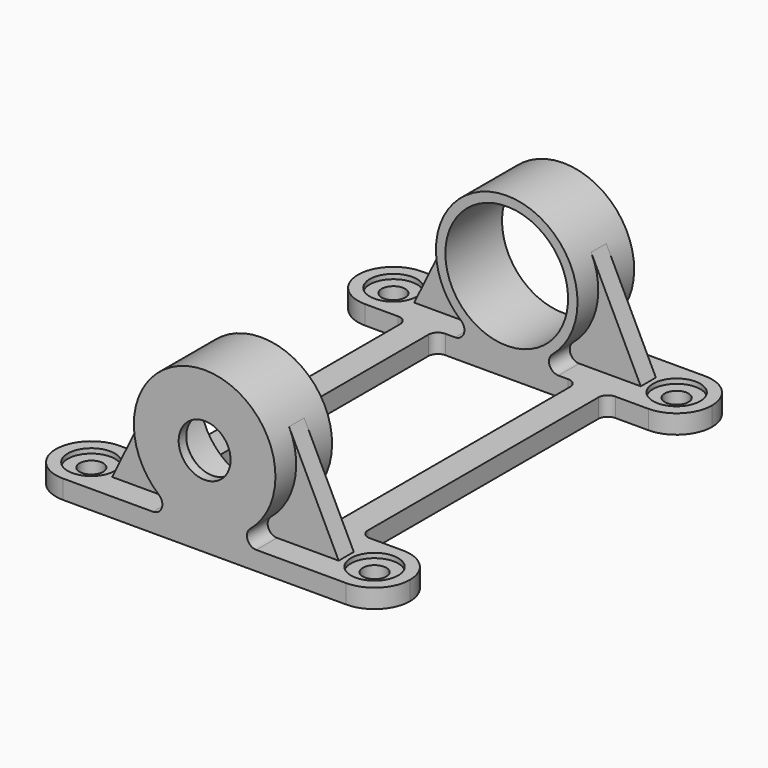
from build123d import *

# Parameters (mm, degrees)
F3_DEPTH       = 7.5
F4_R           = 7.49999
F6_D           = 5
F6_CBORE_D     = 10
F6_CBORE_DEPTH = 1
F8_DEPTH       = 2
F12_R          = 13
F13_DEPTH      = 92
F14_R          = 5.5
F15_DEPTH      = 95.001
F16_W          = 6
F16_H          = 4
F17_DEPTH      = 65
F18_R          = 2
F19_SIZE       = 1


# Not quite as in the source:
# - a fillet or chamfer is up to 0.001 mm smaller than in the source, because OpenCascade refuses the exact size


with BuildPart() as f3:
    # F2 (on Front) → F3 (new body, symmetric)
    with BuildSketch(Plane.XZ):
        with BuildLine():
            Line((-37.5, 0), (0, 0))
            Line((0, 0), (37.5, 0))
            Line((37.5, 0), (37.5, 4))
            Line((37.5, 4), (10.9544511501, 4))
            ThreePointArc((10.9544511501, 4), (9.0757782768, 5.3140056594), (9.6656921913, 7.5294117647))
            ThreePointArc((9.6656921913, 7.5294117647), (14.0900465494, 24.1449575543), (0, 34))
            ThreePointArc((0, 34), (-14.0900465494, 24.1449575543), (-9.6656921913, 7.5294117647))
            ThreePointArc((-9.6656921913, 7.5294117647), (-9.0757782768, 5.3140056594), (-10.9544511501, 4))
            Line((-10.9544511501, 4), (-37.5, 4))
            Line((-37.5, 4), (-37.5, 0))
        make_face()
    extrude(amount=F3_DEPTH, both=True)

    # F4 (radius 7.5 in the source; OpenCascade refuses exactly that, so slightly less here)
    f4_edges = [f3.edges().sort_by_distance(p)[0] for p in [
        (37.5, -7.5, 2),
        (37.5, 7.5, 2),
        (-37.5, -7.5, 2),
        (-37.5, 7.5, 2),
    ]]
    fillet(f4_edges, radius=F4_R)

    # F6 (through all)
    with Locations(Plane.XY.offset(4)):
        with Locations((30, 0), (-30, 0)):
            CounterBoreHole(F6_D / 2, F6_CBORE_D / 2, F6_CBORE_DEPTH)

    # F7 (on Front) → F8 (join, symmetric)
    with BuildSketch(Plane.XZ):
        with BuildLine():
            Line((10.9544511501, 4), (24, 4))
            Line((24, 4), (13.4831460674, 25.5730337079))
            ThreePointArc((13.4831460674, 25.5730337079), (14.6751576274, 15.8952055444), (9.6656921913, 7.5294117647))
            ThreePointArc((9.6656921913, 7.5294117647), (9.0757782768, 5.3140056594), (10.9544511501, 4))
        make_face()
    extrude(amount=F8_DEPTH, both=True)

    # F9: F3 across plane


with BuildPart() as f3_1:
    add(f3.part)
    add(f3.part.mirror(Plane.YZ))


with BuildPart() as f11_1:
    # F11: instance of F3
    add(f3_1.part.mirror(Plane.XZ.offset(40)))


with BuildPart() as f13_tool:
    # F12 (on face) → F13 (new body)
    with BuildSketch(Plane(origin=(0, 7.5, 0), x_dir=(-1, 0, 0), z_dir=(0, 1, 0))):
        with Locations((0, 19)):
            Circle(F12_R)
    extrude(amount=-F13_DEPTH)


with BuildPart() as f3_2:
    add(f3_1.part)

    # F13: cut by f13_tool
    add(f13_tool.part, mode=Mode.SUBTRACT)



with BuildPart() as f11_1_1:
    add(f11_1.part)

    # F13: cut by f13_tool
    add(f13_tool.part, mode=Mode.SUBTRACT)

    # F14 (on face) → F15 (cut, through all)
    with BuildSketch(Plane.XZ.offset(87.5)):
        with Locations((0, 19)):
            Circle(F14_R)
    extrude(amount=-F15_DEPTH, mode=Mode.SUBTRACT)


with BuildPart() as f3_3:
    add(f3_2.part)

    add(f11_1_1.part)  # F17 merges F11_1
    # F16 (on face) → F17 (join, through all)
    with BuildSketch(Plane.XZ.offset(7.5)):
        with Locations((18, 2)):
            Rectangle(F16_W, F16_H)
        with Locations((-18, 2)):
            Rectangle(F16_W, F16_H)
    extrude(amount=F17_DEPTH)

    # F18
    f18_edges = [f3_3.edges().sort_by_distance(p)[0] for p in [
        (21, -7.5, 2),
        (15, -7.5, 2),
        (21, -72.5, 2),
        (15, -72.5, 2),
        (-21, -7.5, 2),
        (-21, -72.5, 2),
        (-15, -72.5, 2),
        (-15, -7.5, 2),
    ]]
    fillet(f18_edges, radius=F18_R)

    # F19
    f19_edges = [f3_3.edges().sort_by_distance(p)[0] for p in [
        (-5.5, -84.5, 19),
    ]]
    chamfer(f19_edges, length=F19_SIZE)


solid = f3_3.part
